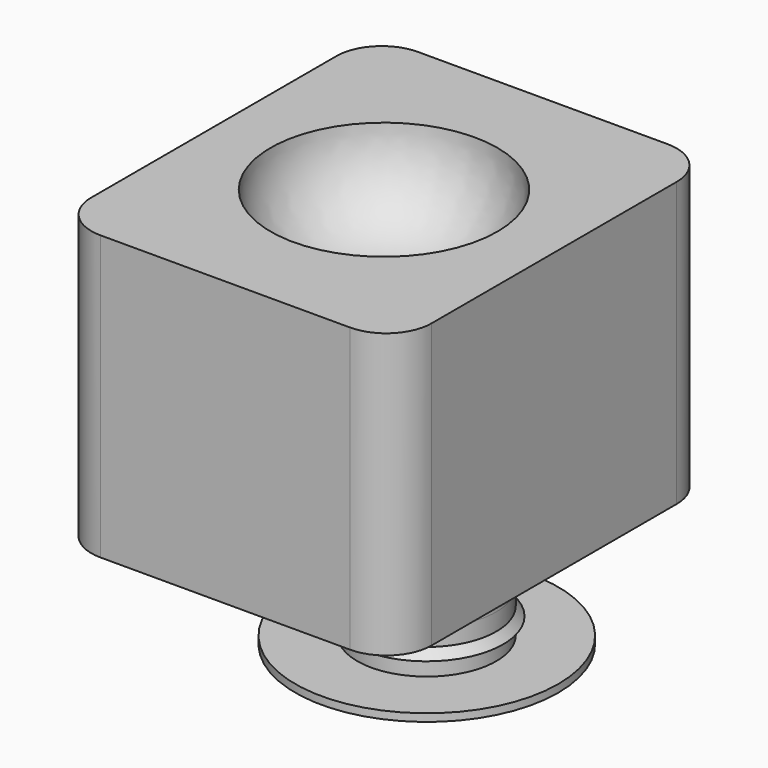
from build123d import *

# Parameters (mm, degrees)
F2_W     = 70
F2_H     = 50
F3_DEPTH = 30
F4_R     = 8
F6_R     = 20
F7_DEPTH = 15.7


# Not quite as in the source:
# - a fillet or chamfer that OpenCascade refuses, or shapes differently, is made with other operations: its cross-section is extruded or revolved along the edge and cut away or added


with BuildPart() as f1:
    # F0 (on Front) → F1 (revolve)
    with BuildSketch(Plane.XZ):
        with BuildLine():
            Line((-23.175, 0), (0, 0))
            Line((0, 0), (0, 35))
            Line((0, 35), (-1.88, 35))
            Line((-1.88, 35), (-3.88, 35))
            Line((-3.88, 35), (-3.88, 28.2))
            Line((-3.88, 28.2), (-3.95, 28.2))
            ThreePointArc((-3.95, 28.2), (-4.5863961031, 27.9363961031), (-4.85, 27.3))
            Line((-4.85, 27.3), (-4.85, 27.1))
            Line((-4.85, 27.1), (-4.85, 26.9))
            ThreePointArc((-4.85, 26.9), (-4.5863961031, 26.2636038969), (-3.95, 26))
            Line((-3.95, 26), (-3.88, 26))
            Line((-3.88, 26), (-3.88, 16))
            Line((-3.88, 16), (-5.25, 16))
            ThreePointArc((-5.25, 16), (-10.1997474683, 13.9497474683), (-12.25, 9))
            Line((-12.25, 9), (-12.25, 5.95))
            Line((-12.25, 5.95), (-12.25, 4.35))
            Line((-12.25, 4.35), (-12.25, 1.35))
            Line((-12.25, 1.35), (-13.46, 1.35))
            Line((-13.46, 1.35), (-23.175, 1.35))
            Line((-23.175, 1.35), (-23.175, 0))
        make_face()
        Polygon((-13.46, 4.35), (-13.46, 1.35), (-12.25, 1.35), (-12.25, 4.35), (-12.25, 5.95), align=None)
        with BuildLine():
            Line((-4.85, 26.9), (-5.25, 16))
            Line((-5.25, 16), (-3.88, 16))
            Line((-3.88, 16), (-3.88, 26))
            Line((-3.88, 26), (-3.95, 26))
            ThreePointArc((-3.95, 26), (-4.5863961031, 26.2636038969), (-4.85, 26.9))
        make_face()
    revolve(axis=Axis((0, 0, 17.5), (0, 0, 1)))


with BuildPart() as f3:
    # F2 (on Right) → F3 (new body, symmetric)
    with BuildSketch(Plane.YZ):
        with Locations((0, 25)):
            Rectangle(F2_W, F2_H)
    extrude(amount=F3_DEPTH, both=True)

    # F4
    f4_edges = [f3.edges().sort_by_distance(p)[0] for p in [
        (30, -35, 25),
        (30, 35, 25),
        (-30, -35, 25),
        (-30, 35, 25),
    ]]
    fillet(f4_edges, radius=F4_R)

    # F5: cut F1
    add(f1.part, mode=Mode.SUBTRACT)

    # F6 (on face) → F7 (cut)
    with BuildSketch(Plane.XY.offset(50)):
        Circle(F6_R)
    extrude(amount=-F7_DEPTH, mode=Mode.SUBTRACT)

    # F8: fillet of radius 15.9338095117 on 1 edges, made by hand

    # F8_s1 → F8_t2 (revolve)
    with BuildSketch(Plane.XZ):
        with BuildLine():
            ThreePointArc((20, 50), (15.251841133, 38.8845416548), (4.0679060175, 34.3))
            Line((4.0679060175, 34.3), (20, 34.3))
            Line((20, 34.3), (20, 50))
        make_face()
    revolve(axis=Axis((0, 0, 34.3), (0, 0, 1)))


with BuildPart() as f10:
    # F9 (on Front) → F10 (revolve)
    with BuildSketch(Plane.XZ):
        with BuildLine():
            Line((-15.6303802583, -18.0891831181), (6.1008301564, -18.0891831181))
            Line((6.1008301564, -18.0891831181), (6.1008301564, 16.9108168819))
            Line((6.1008301564, 16.9108168819), (5.6646197417, 16.9108168819))
            ThreePointArc((5.6646197417, 16.9108168819), (4.2504061793, 16.3250304443), (3.6646197417, 14.9108168819))
            Line((3.6646197417, 14.9108168819), (3.6646197417, 9.9108168819))
            Line((3.6646197417, 9.9108168819), (3.5946197417, 9.9108168819))
            ThreePointArc((3.5946197417, 9.9108168819), (2.9582236386, 9.647212985), (2.6946197417, 9.0108168819))
            Line((2.6946197417, 9.0108168819), (2.6946197417, 8.8108168819))
            ThreePointArc((2.6946197417, 8.8108168819), (2.9582236386, 8.1744207789), (3.5946197417, 7.9108168819))
            Line((3.5946197417, 7.9108168819), (3.6646197417, 7.9108168819))
            Line((3.6646197417, 7.9108168819), (3.6646197417, -2.0891831181))
            Line((3.6646197417, -2.0891831181), (2.2946197417, -2.0891831181))
            ThreePointArc((2.2946197417, -2.0891831181), (-2.6551277266, -4.1394356497), (-4.7053802583, -9.0891831181))
            Line((-4.7053802583, -9.0891831181), (-4.7053802583, -12.1391831181))
            Line((-4.7053802583, -12.1391831181), (-5.9153802583, -13.7391831181))
            Line((-5.9153802583, -13.7391831181), (-4.7053802583, -13.7391831181))
            Line((-4.7053802583, -13.7391831181), (-4.7053802583, -16.7391831181))
            Line((-4.7053802583, -16.7391831181), (-15.6303802583, -16.7391831181))
            Line((-15.6303802583, -16.7391831181), (-15.6303802583, -18.0891831181))
        make_face()
    revolve(axis=Axis((7.5446197417, 0, -0.5891831181), (0, 0, 1)))


solid = Compound([f1.part, f3.part, f10.part])
